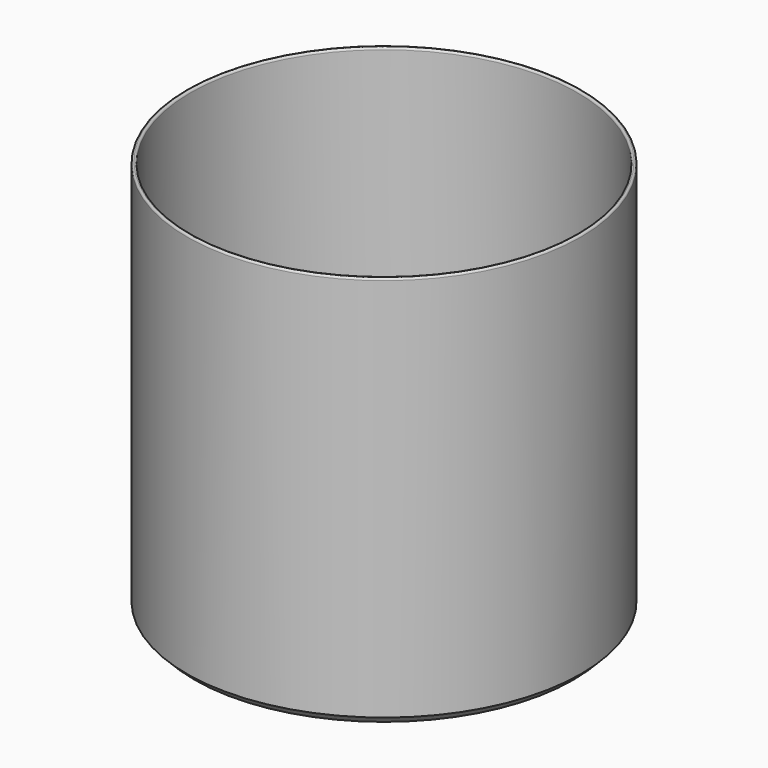
from build123d import *

# Parameters (mm, degrees)
F0_R     = 50
F1_DEPTH = 50
F2_DEPTH = 50
F3_SIZE  = 2
F4_T     = -1
F5_R     = 0.49999


# Not quite as in the source:
# - a fillet or chamfer is up to 0.001 mm smaller than in the source, because OpenCascade refuses the exact size


with BuildPart() as f1:
    # F0 (on Top) → F1 (new body)
    with BuildSketch(Plane.XY):
        Circle(F0_R)
    extrude(amount=F1_DEPTH)

    # F2 (add): a face of the model
    f2_faces = [f1.faces().sort_by_distance(p)[0] for p in [
        (0, 0, 0),
    ]]
    extrude(f2_faces, amount=F2_DEPTH)

    # F3
    f3_edges = [f1.edges().sort_by_distance(p)[0] for p in [
        (-50, 0, -50),
    ]]
    chamfer(f3_edges, length=F3_SIZE)

    # F4
    f4_openings = [f1.faces().sort_by_distance(p)[0] for p in [
        (0, 0, 50),
    ]]
    offset(amount=F4_T, openings=f4_openings)

    # F5 (radius 0.5 in the source; OpenCascade refuses exactly that, so slightly less here)
    f5_edges = [f1.edges().sort_by_distance(p)[0] for p in [
        (-50, 0, 50),
        (-49, 0, 50),
    ]]
    fillet(f5_edges, radius=F5_R)


solid = f1.part
